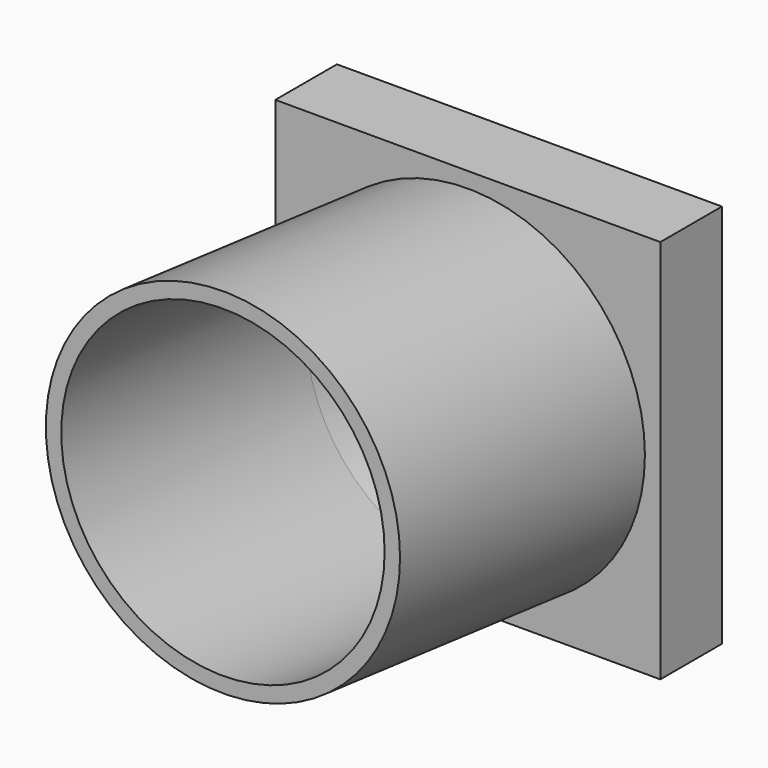
from build123d import *

# Parameters (mm, degrees)
F1_R     = 11.5
F1_R_2   = 10.5
F0_W     = 25
F0_H     = 25
F4_DEPTH = 5
F5_R     = 10.5
F6_DEPTH = 5.001


with BuildPart() as f3:
    # F3: sweep along a path in F2
    with BuildLine(Plane.YZ) as f3_path:
        Line((0, 8.3436881795), (-19.8769871225, 10.5584980885))
    # F1 (on face) → F3 (sweep)
    with BuildSketch(Plane.XZ):
        with Locations((-7.256067358, 8.3436881795)):
            Circle(F1_R)
        with Locations((-7.256067358, 8.3436881795)):
            Circle(F1_R_2, mode=Mode.SUBTRACT)
    sweep(path=f3_path.line)

    # F0 (on Front) → F4 (join)
    with BuildSketch(Plane.XZ):
        with Locations((-7.256067358, 8.3436881795)):
            Rectangle(F0_W, F0_H)
    extrude(amount=-F4_DEPTH)

    # F5 (on face) → F6 (cut, through all)
    with BuildSketch(Plane.XZ):
        with Locations((-7.256067358, 8.3436881795)):
            Circle(F5_R)
    extrude(amount=-F6_DEPTH, mode=Mode.SUBTRACT)


solid = f3.part
